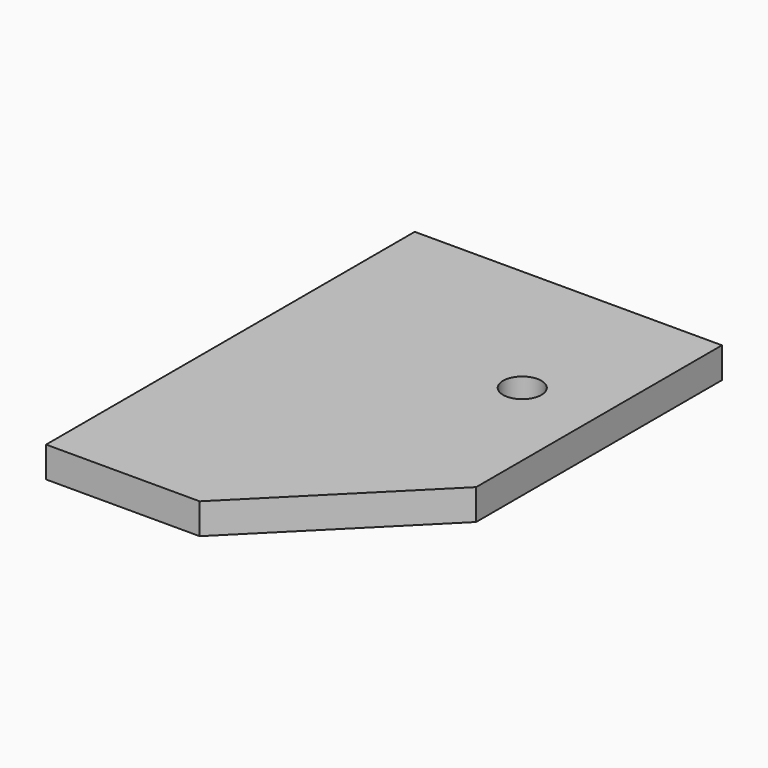
from build123d import *

# Parameters (mm, degrees)
F0_R     = 5
F1_DEPTH = 8


# Not quite as in the source:
# - a feature names something its author has since deleted; it is built from what else it names


with BuildPart() as f1:
    # F0 (on Top) → F1 (new body)
    with BuildSketch(Plane.XY):
        Polygon((40, 20), (40, 60), (-40, 60), (-40, -60), (0, -60), (40, -20), align=None)
        with Locations((20, 20)):
            Circle(F0_R, mode=Mode.SUBTRACT)
    extrude(amount=F1_DEPTH)


solid = f1.part
